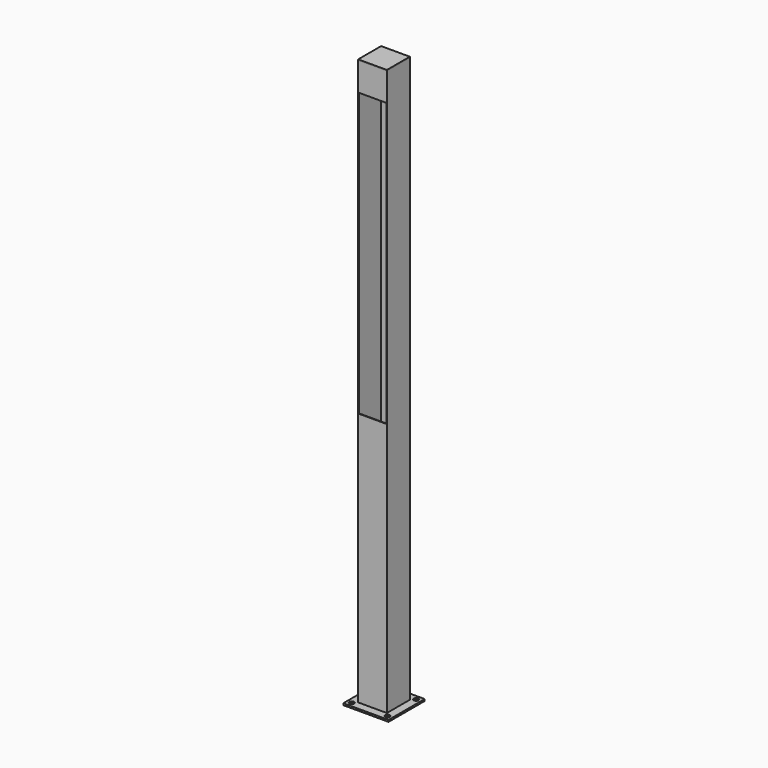
from build123d import *

# Parameters (mm, degrees)
F0_W      = 152.4
F0_H      = 152.4
F0_W_2    = 146
F0_H_2    = 146
F1_DEPTH  = 3000
F2_W      = 146
F2_H      = 1500
F3_DEPTH  = 148.8
F6_W      = 152.4
F6_H      = 152.4
F6_W_2    = 146
F6_H_2    = 146
F7_DEPTH  = 4.762
F8_W      = 240
F8_H      = 240
F9_DEPTH  = 9.5
F10_R     = 12.7
F11_DEPTH = 9.5


# Not quite as in the source:
# - the program builds the solid bodies; features that only make, move or delete a surface that nothing else refers to are left out


with BuildPart() as f1:
    # F0 (on Top) → F1 (new body)
    with BuildSketch(Plane.XY):
        Rectangle(F0_W, F0_H)
        Rectangle(F0_W_2, F0_H_2, mode=Mode.SUBTRACT)
    extrude(amount=F1_DEPTH)

    # F2 (on face) → F3 (cut)
    with BuildSketch(Plane.XZ.offset(76.2)):
        with Locations((0, 2100)):
            Rectangle(F2_W, F2_H)
    extrude(amount=-F3_DEPTH, mode=Mode.SUBTRACT)


with BuildPart() as f7:
    # F6 (on face) → F7 (new body)
    with BuildSketch(Plane.XY.offset(3000)):
        Rectangle(F6_W, F6_H)
        Rectangle(F6_W_2, F6_H_2, mode=Mode.SUBTRACT)
        Rectangle(F6_W_2, F6_H_2)
    extrude(amount=F7_DEPTH)


with BuildPart() as f9:
    # F8 (on face) → F9 (new body)
    with BuildSketch(Plane(origin=(0, 0, 0), x_dir=(1, 0, 0), z_dir=(0, 0, -1))):
        Rectangle(F8_W, F8_H)
    extrude(amount=F9_DEPTH)

    # F10 (on face) → F11 (cut, through all)
    with BuildSketch(Plane(origin=(0, 0, -9.5), x_dir=(1, 0, 0), z_dir=(0, 0, -1))):
        with Locations((-95, 95)):
            Circle(F10_R)
        with Locations((-95, -95)):
            Circle(F10_R)
        with Locations((95, 95)):
            Circle(F10_R)
        with Locations((95, -95)):
            Circle(F10_R)
        Circle(F10_R)
    extrude(amount=-F11_DEPTH, mode=Mode.SUBTRACT)


solid = Compound([f1.part, f7.part, f9.part])
